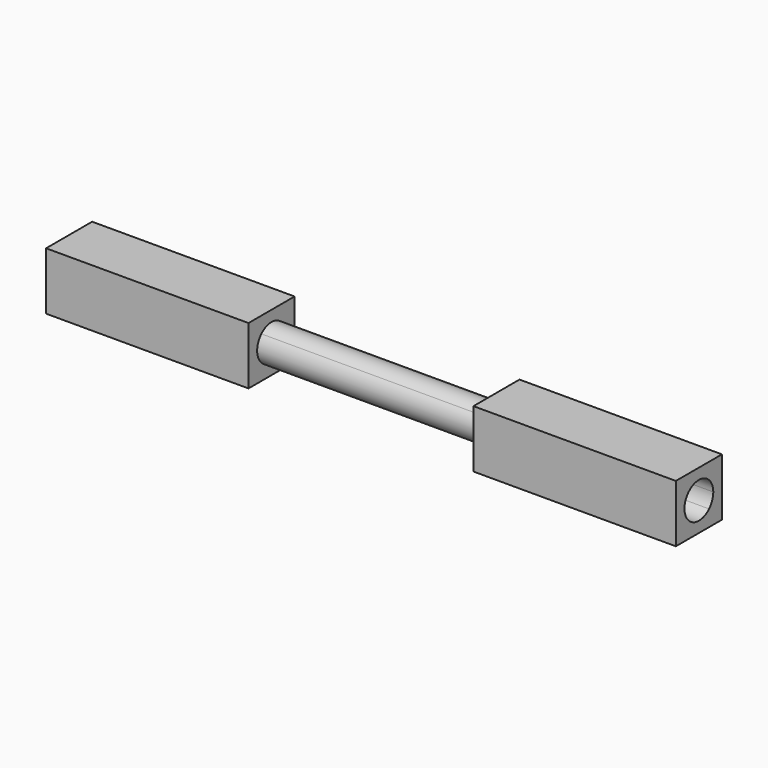
from build123d import *

# Parameters (mm, degrees)
F1_DEPTH = 35
F2_DEPTH = 12.5
F3_DEPTH = 12.5


with BuildPart() as f1:
    # F0 (on Right) → F1 (new body, symmetric)
    with BuildSketch(Plane.YZ):
        with BuildLine():
            Line((-1.414214, -1.414214), (-3.2, -3.2))
            Line((-3.2, -3.2), (3.2, -3.2))
            Line((3.2, -3.2), (1.414214, -1.414214))
            ThreePointArc((1.414214, -1.414214), (0, -2), (-1.414214, -1.414214))
        make_face()
        with BuildLine():
            Line((-1.414214, 1.414214), (-3.2, 3.2))
            Line((-3.2, 3.2), (-3.2, -3.2))
            Line((-3.2, -3.2), (-1.414214, -1.414214))
            ThreePointArc((-1.414214, -1.414214), (-2, 0), (-1.414214, 1.414214))
        make_face()
        with BuildLine():
            Line((3.2, -3.2), (3.2, 3.2))
            Line((3.2, 3.2), (1.414214, 1.414214))
            ThreePointArc((1.414214, 1.414214), (1.847759, 0.765367), (2, 0))
            ThreePointArc((2, 0), (1.847759, -0.765367), (1.414214, -1.414214))
            Line((1.414214, -1.414214), (3.2, -3.2))
        make_face()
        with BuildLine():
            Line((3.2, 3.2), (-3.2, 3.2))
            Line((-3.2, 3.2), (-1.414214, 1.414214))
            ThreePointArc((-1.414214, 1.414214), (0, 2), (1.414214, 1.414214))
            Line((1.414214, 1.414214), (3.2, 3.2))
        make_face()
    extrude(amount=F1_DEPTH, both=True)

    # F0 (on Right) → F3 (cut, symmetric)
    with BuildSketch(Plane.YZ):
        with BuildLine():
            Line((3.2, 3.2), (-3.2, 3.2))
            Line((-3.2, 3.2), (-1.414214, 1.414214))
            ThreePointArc((-1.414214, 1.414214), (0, 2), (1.414214, 1.414214))
            Line((1.414214, 1.414214), (3.2, 3.2))
        make_face()
        with BuildLine():
            Line((-1.414214, 1.414214), (-3.2, 3.2))
            Line((-3.2, 3.2), (-3.2, -3.2))
            Line((-3.2, -3.2), (-1.414214, -1.414214))
            ThreePointArc((-1.414214, -1.414214), (-2, 0), (-1.414214, 1.414214))
        make_face()
        with BuildLine():
            Line((-1.414214, -1.414214), (-3.2, -3.2))
            Line((-3.2, -3.2), (3.2, -3.2))
            Line((3.2, -3.2), (1.414214, -1.414214))
            ThreePointArc((1.414214, -1.414214), (0, -2), (-1.414214, -1.414214))
        make_face()
        with BuildLine():
            Line((3.2, -3.2), (3.2, 3.2))
            Line((3.2, 3.2), (1.414214, 1.414214))
            ThreePointArc((1.414214, 1.414214), (1.847759, 0.765367), (2, 0))
            ThreePointArc((2, 0), (1.847759, -0.765367), (1.414214, -1.414214))
            Line((1.414214, -1.414214), (3.2, -3.2))
        make_face()
    extrude(amount=F3_DEPTH, both=True, mode=Mode.SUBTRACT)


with BuildPart() as f2:
    # F0 (on Right) → F2 (new body, symmetric)
    with BuildSketch(Plane.YZ):
        with BuildLine():
            ThreePointArc((1.414214, 1.414214), (0, 2), (-1.414214, 1.414214))
            Line((-1.414214, 1.414214), (0, 0))
            Line((0, 0), (1.414214, 1.414214))
        make_face()
        with BuildLine():
            ThreePointArc((2, 0), (1.847759, 0.765367), (1.414214, 1.414214))
            Line((1.414214, 1.414214), (0, 0))
            Line((0, 0), (1.414214, -1.414214))
            ThreePointArc((1.414214, -1.414214), (1.847759, -0.765367), (2, 0))
        make_face()
        with BuildLine():
            Line((0, 0), (-1.414214, -1.414214))
            ThreePointArc((-1.414214, -1.414214), (0, -2), (1.414214, -1.414214))
            Line((1.414214, -1.414214), (0, 0))
        make_face()
        with BuildLine():
            Line((0, 0), (-1.414214, 1.414214))
            ThreePointArc((-1.414214, 1.414214), (-2, 0), (-1.414214, -1.414214))
            Line((-1.414214, -1.414214), (0, 0))
        make_face()
    extrude(amount=F2_DEPTH, both=True)


solid = Compound([f1.part, f2.part])
